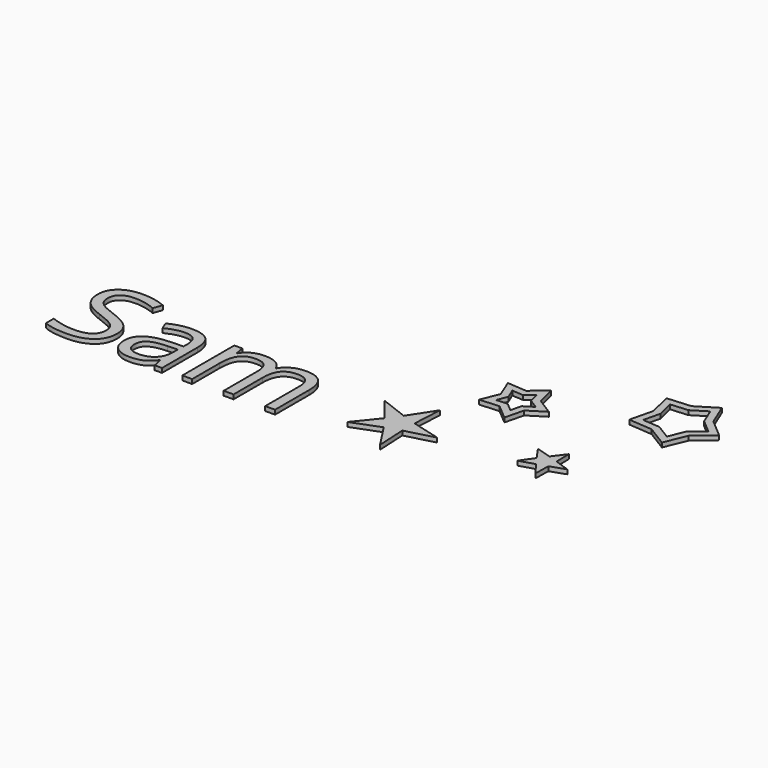
from build123d import *

# Parameters (mm, degrees)
F0_TEXT_SIZE = 13.8688955963
F1_DEPTH     = 0.5


# Not quite as in the source:
# - Text() gives the source's letters only with a copy of the font that has no kerning and outlines rounded to 1/6400 em; it was checked with that copy


with BuildPart() as f1:
    # F0 (on Top) → F1 (new body)
    with BuildSketch(Plane.XY):
        Polygon((45.5197678753, 19.2148680571), (42.8062423837, 19.0067321436), (43.4468188584, 16.3616985083), (42.8062423837, 13.7166648729), (45.5197678753, 13.5085289594), (47.8373953331, 12.0819441849), (48.8738698415, 14.5983427514), (50.9468188584, 16.3616985083), (48.8738698415, 18.1250542651), (47.8373953331, 20.6414528316), align=None)
        Polygon((47.4558552841, 19.467193304), (48.2079466306, 17.641232732), (49.7121293236, 16.3616985083), (48.2079466306, 15.0821642845), (47.4558552841, 13.2562037126), (45.7741279079, 14.2913686445), (43.8051272001, 14.4423971726), (44.2699452149, 16.3616985083), (43.8051272001, 18.2809998439), (45.7741279079, 18.4320283721), align=None, mode=Mode.SUBTRACT)
        Polygon((32.15595247, 12.3196945685), (29.9424269785, 12.4748299189), (30.7739864588, 10.4175815359), (29.9424269785, 8.3603331529), (32.15595247, 8.5154685033), (33.8555459391, 7.0888837288), (34.3920204475, 9.2420110313), (36.2739864588, 10.4175815359), (34.3920204475, 11.5931520405), (33.8555459391, 13.7462793429), align=None)
        Polygon((33.3889164299, 12.3101413844), (33.6939336388, 11.0859622857), (34.7639416466, 10.4175815359), (33.6939336388, 9.7492007861), (33.3889164299, 8.5250216874), (32.4225979039, 9.3361187653), (31.1640788938, 9.2479152238), (31.6368692086, 10.4175815359), (31.1640788938, 11.587247848), (32.4225979039, 11.4990443064), align=None, mode=Mode.SUBTRACT)
        Polygon((41.6785921238, 3.7183704865), (39.9650666323, 4.236777101), (40.9876091182, 2.7673139703), (39.9650666323, 1.2978508395), (41.6785921238, 1.816257454), (42.7601516042, 0.3896726795), (42.7966261126, 2.179528718), (44.4876091182, 2.7673139703), (42.7966261126, 3.3550992225), (42.7601516042, 5.144955261), align=None)
        Polygon((26.6473156337, 1.7384390408), (23.4702646506, 2.9568879016), (25.6108411252, 0.3118542663), (23.4702646506, -2.333179369), (26.6473156337, -1.1147305081), (28.5014175999, -3.967900057), (28.3243666168, -0.5698236121), (31.6108411252, 0.3118542663), (28.3243666168, 1.1935321448), (28.5014175999, 4.5916085897), align=None)
        with Locations((-10.1407284383, -4.5150844783)):
            Text('Sam', F0_TEXT_SIZE, font='Open Sans', text_align=(TextAlign.LEFT, TextAlign.BOTTOM))
    extrude(amount=F1_DEPTH)


solid = f1.part
